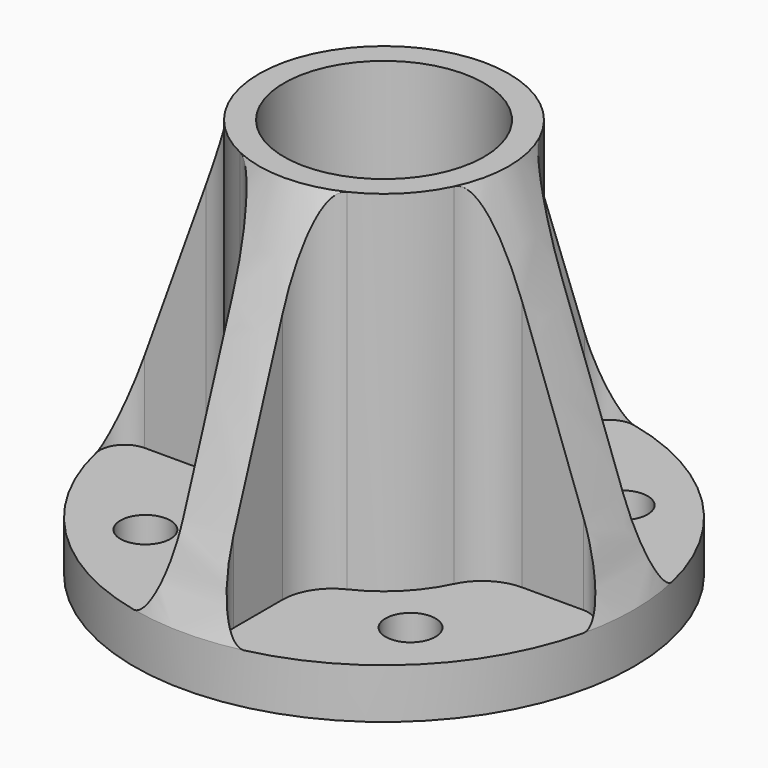
from build123d import *

# Parameters (mm, degrees)
F0_R            = 63.5
F1_DEPTH        = 12.7
F2_R            = 31.75
F3_DEPTH        = 88.9
F7_DEPTH        = 88.9010001
F8_R            = 6.35
F9_DEPTH        = 12.701
F9_COPIES_COUNT = 4
F10_R           = 25.4
F11_DEPTH       = 101.601


# Not quite as in the source:
# - a pattern or mirror of a feature is missing from the dataset's text; its kind, count and spacing are read off the source's solid


with BuildPart() as f1:
    # F0 (on Top) → F1 (new body)
    with BuildSketch(Plane.XY):
        Circle(F0_R)
    extrude(amount=F1_DEPTH)

    # F2 (on face) → F3 (join)
    with BuildSketch(Plane.XY.offset(12.7)):
        Circle(F2_R)
    extrude(amount=F3_DEPTH)

    # F4 (on Right) → F5 (revolve)
    with BuildSketch(Plane.YZ):
        Polygon((-31.75, 12.7), (-31.75, 101.6), (-63.5, 12.7), align=None)
    revolve(axis=Axis((0, 0, 73.5445022583), (0, 0, 1)))

    # F6 (on face) → F7 (cut, through all)
    with BuildSketch(Plane.XY.offset(12.7)):
        with BuildLine():
            ThreePointArc((-14.1111111111, 61.9122487333), (-44.9012806053, 44.9012806053), (-61.9122487333, 14.1111111111))
            ThreePointArc((-61.9122487333, 14.1111111111), (-60.6850472058, 8.7400792657), (-55.7210238599, 6.35))
            Line((-55.7210238599, 6.35), (-40.1609262841, 6.35))
            ThreePointArc((-40.1609262841, 6.35), (-33.3724907396, 8.3165409649), (-28.6863759172, 13.6071428571))
            ThreePointArc((-28.6863759172, 13.6071428571), (-22.4506403027, 22.4506403027), (-13.6071428571, 28.6863759172))
            ThreePointArc((-13.6071428571, 28.6863759172), (-8.3165409649, 33.3724907396), (-6.35, 40.1609262841))
            Line((-6.35, 40.1609262841), (-6.35, 55.7210238599))
            ThreePointArc((-6.35, 55.7210238599), (-8.7400792657, 60.6850472058), (-14.1111111111, 61.9122487333))
        make_face()
        with BuildLine():
            Line((-40.1609262841, -6.35), (-55.7210238599, -6.35))
            ThreePointArc((-55.7210238599, -6.35), (-60.6850472058, -8.7400792657), (-61.9122487333, -14.1111111111))
            ThreePointArc((-61.9122487333, -14.1111111111), (-44.9012806053, -44.9012806053), (-14.1111111111, -61.9122487333))
            ThreePointArc((-14.1111111111, -61.9122487333), (-8.7400792657, -60.6850472058), (-6.35, -55.7210238599))
            Line((-6.35, -55.7210238599), (-6.35, -40.1609262841))
            ThreePointArc((-6.35, -40.1609262841), (-8.3165409649, -33.3724907396), (-13.6071428571, -28.6863759172))
            ThreePointArc((-13.6071428571, -28.6863759172), (-22.4506403027, -22.4506403027), (-28.6863759172, -13.6071428571))
            ThreePointArc((-28.6863759172, -13.6071428571), (-33.3724907396, -8.3165409649), (-40.1609262841, -6.35))
        make_face()
        with BuildLine():
            Line((6.35, -40.1609262841), (6.35, -55.7210238599))
            ThreePointArc((6.35, -55.7210238599), (8.7400792657, -60.6850472058), (14.1111111111, -61.9122487333))
            ThreePointArc((14.1111111111, -61.9122487333), (44.9012806053, -44.9012806053), (61.9122487333, -14.1111111111))
            ThreePointArc((61.9122487333, -14.1111111111), (60.6850472058, -8.7400792657), (55.7210238599, -6.35))
            Line((55.7210238599, -6.35), (40.1609262841, -6.35))
            ThreePointArc((40.1609262841, -6.35), (33.3724907396, -8.3165409649), (28.6863759172, -13.6071428571))
            ThreePointArc((28.6863759172, -13.6071428571), (22.4506403027, -22.4506403027), (13.6071428571, -28.6863759172))
            ThreePointArc((13.6071428571, -28.6863759172), (8.3165409649, -33.3724907396), (6.35, -40.1609262841))
        make_face()
        with BuildLine():
            Line((40.1609262841, 6.35), (55.7210238599, 6.35))
            ThreePointArc((55.7210238599, 6.35), (60.6850472058, 8.7400792657), (61.9122487333, 14.1111111111))
            ThreePointArc((61.9122487333, 14.1111111111), (44.9012806053, 44.9012806053), (14.1111111111, 61.9122487333))
            ThreePointArc((14.1111111111, 61.9122487333), (8.7400792657, 60.6850472058), (6.35, 55.7210238599))
            Line((6.35, 55.7210238599), (6.35, 40.1609262841))
            ThreePointArc((6.35, 40.1609262841), (8.3165409649, 33.3724907396), (13.6071428571, 28.6863759172))
            ThreePointArc((13.6071428571, 28.6863759172), (22.4506403027, 22.4506403027), (28.6863759172, 13.6071428571))
            ThreePointArc((28.6863759172, 13.6071428571), (33.3724907396, 8.3165409649), (40.1609262841, 6.35))
        make_face()
    extrude(amount=F7_DEPTH, mode=Mode.SUBTRACT)

    # F8 (on face) → F9 (cut, through all)
    with BuildSketch(Plane.XY.offset(12.7)):
        with Locations((-33.675960454, 33.675960454)):
            Circle(F8_R)
    f9 = extrude(amount=-F9_DEPTH, mode=Mode.SUBTRACT)

    # F9_copies: F9 ×4 about axis
    f9_copies_axis = Axis((0, 0, 0), (0, 0, 1))
    for i in range(1, F9_COPIES_COUNT):
        add(f9.rotate(f9_copies_axis, i * 360 / F9_COPIES_COUNT), mode=Mode.SUBTRACT)

    # F10 (on face) → F11 (cut, through all)
    with BuildSketch(Plane.XY.offset(101.6)):
        Circle(F10_R)
    extrude(amount=-F11_DEPTH, mode=Mode.SUBTRACT)


solid = f1.part
